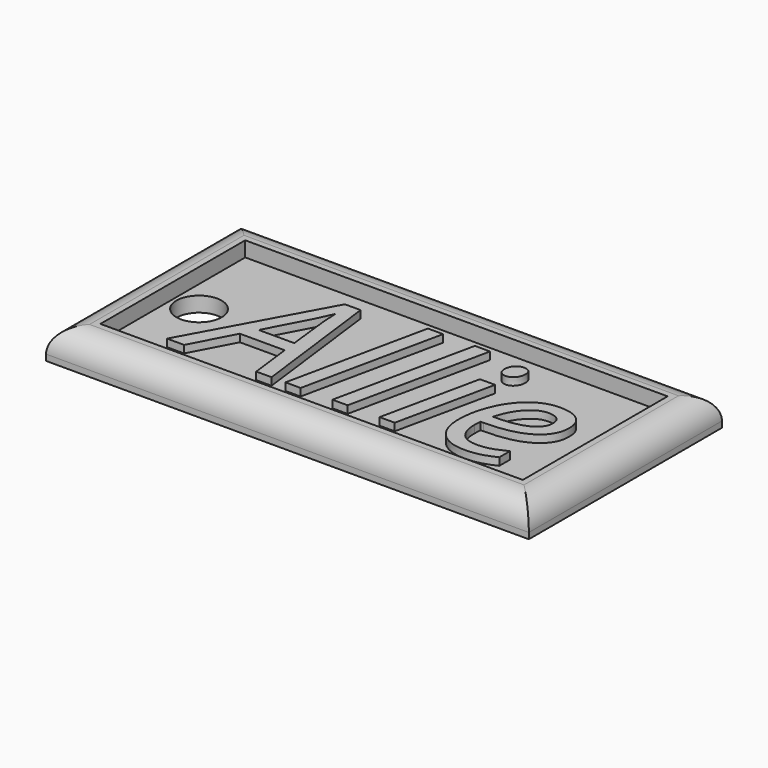
from build123d import *

# Parameters (mm, degrees)
F0_W         = 44.45
F0_H         = 19.05
F0_R         = 2.38125
F1_DEPTH     = 1.5875
F0_W_2       = 50.8
F0_H_2       = 25.4
F2_DEPTH     = 3.175
F3_TEXT_SIZE = 19.4671537934
F4_DEPTH     = 0.79375
F5_R         = 2.54


# Not quite as in the source:
# - a length typed as a fraction of an inch, garbled in the dataset ("3 / 203.2 mm" for 3/8 in), is restored
# - Text() gives the source's letters only with a copy of the font that has no kerning and outlines rounded to 1/6400 em; it was checked with that copy


with BuildPart() as f1:
    # F0 (on Top) → F1 (new body)
    with BuildSketch(Plane.XY):
        with Locations((25.4, 12.7)):
            Rectangle(F0_W, F0_H)
        with Locations((5.9374803677, 12.7)):
            Circle(F0_R, mode=Mode.SUBTRACT)
    extrude(amount=F1_DEPTH)

    # F0 (on Top) → F2 (join)
    with BuildSketch(Plane.XY):
        with Locations((25.4, 12.7)):
            Rectangle(F0_W_2, F0_H_2)
        with Locations((25.4, 12.7)):
            Rectangle(F0_W, F0_H, mode=Mode.SUBTRACT)
    extrude(amount=F2_DEPTH)

    # F3 (on face) → F4 (join)
    with BuildSketch(Plane.XY.offset(1.5875)):
        with Locations((9.2468978837, 5.7428106666)):
            Text('Allie', F3_TEXT_SIZE, font='Open Sans', font_style=FontStyle.ITALIC, text_align=(TextAlign.LEFT, TextAlign.BOTTOM))
    extrude(amount=F4_DEPTH)

    # F5
    f5_edges = [f1.edges().sort_by_distance(p)[0] for p in [
        (25.4, 0, 3.175),
        (0, 12.7, 3.175),
        (25.4, 25.4, 3.175),
        (50.8, 12.7, 3.175),
    ]]
    fillet(f5_edges, radius=F5_R)


solid = f1.part
